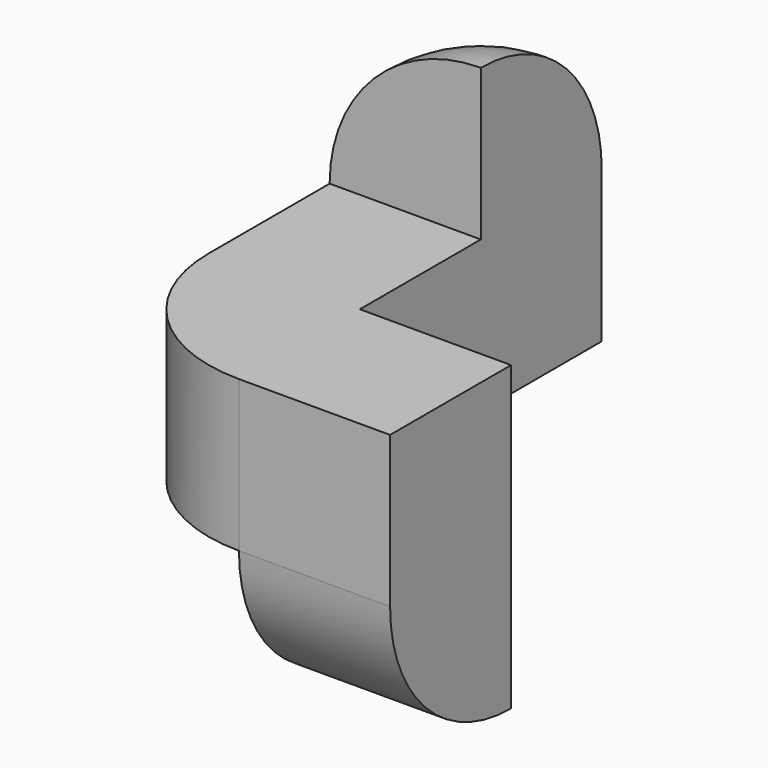
from build123d import *

# Parameters (mm, degrees)
F0_W     = 25.4
F0_H     = 25.4
F1_DEPTH = 25.4
F2_W     = 25.4
F2_H     = 25.4
F3_DEPTH = 25.4
F4_W     = 25.4
F4_H     = 25.4
F5_DEPTH = 25.4
F6_R     = 25.39999


# Not quite as in the source:
# - a fillet or chamfer is up to 0.001 mm smaller than in the source, because OpenCascade refuses the exact size


with BuildPart() as f1:
    # F0 (on Top) → F1 (new body)
    with BuildSketch(Plane.XY):
        with Locations((12.7, 12.7)):
            Rectangle(F0_W, F0_H)
    extrude(amount=F1_DEPTH)

    # F2 (on face) → F3 (join)
    with BuildSketch(Plane.XY.offset(25.4)):
        Polygon((-25.4, 0), (0, 0), (0, 25.4), (0, 76.2), (-25.4, 76.2), align=None)
        with Locations((12.7, 12.7)):
            Rectangle(F2_W, F2_H)
    extrude(amount=F3_DEPTH)

    # F4 (on face) → F5 (join)
    with BuildSketch(Plane.XY.offset(50.8)):
        with Locations((-12.7, 63.5)):
            Rectangle(F4_W, F4_H)
    extrude(amount=F5_DEPTH)

    # F6 (radius 25.4 in the source; OpenCascade refuses exactly that, so slightly less here)
    f6_edges = [f1.edges().sort_by_distance(p)[0] for p in [
        (12.7, 0, 0),
        (-25.4, 0, 38.1),
        (-25.4, 63.5, 76.2),
        (-12.7, 76.2, 76.2),
        (-25.4, 76.2, 50.8),
    ]]
    fillet(f6_edges, radius=F6_R)


solid = f1.part
